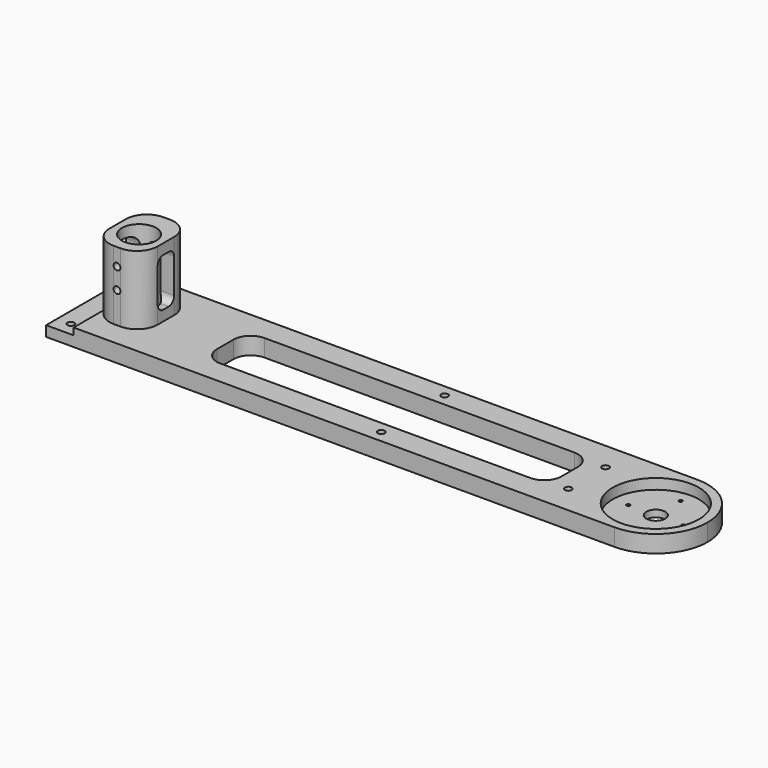
from build123d import *

# Parameters (mm, degrees)
F0_W      = 180
F0_H      = 30
F0_R      = 1
F0_W_2    = 100
F0_H_2    = 16
F1_DEPTH  = 5
F2_R      = 12.5
F2_R_2    = 0.5
F2_R_3    = 2.75
F3_DEPTH  = 3
F4_DEPTH  = 25
F5_R      = 14.99999
F2_R_4    = 5
F6_DEPTH  = 25
F7_R      = 5
F2_W      = 14
F2_H      = 18
F8_DEPTH  = 20
F9_R      = 6
F2_R_5    = 1
F10_DEPTH = 2
F11_W     = 6
F11_H     = 14
F12_DEPTH = 25
F13_R     = 2
F15_DEPTH = 25


# Not quite as in the source:
# - a fillet or chamfer is up to 0.001 mm smaller than in the source, because OpenCascade refuses the exact size


with BuildPart() as f1:
    # F0 (on Top) → F1 (new body)
    with BuildSketch(Plane.XY):
        with Locations((10, -11.8972941886)):
            Rectangle(F0_W, F0_H)
        with Locations((-76, -22.8972941886)):
            Circle(F0_R, mode=Mode.SUBTRACT)
        with Locations((14.5, -23.3972941886)):
            Circle(F0_R, mode=Mode.SUBTRACT)
        with Locations((10, -11.8972941886)):
            Rectangle(F0_W_2, F0_H_2, mode=Mode.SUBTRACT)
        with Locations((65, -18.6472941886)):
            Circle(F0_R, mode=Mode.SUBTRACT)
        with Locations((-76, -0.8972941886)):
            Circle(F0_R, mode=Mode.SUBTRACT)
        with Locations((65, -5.1472941886)):
            Circle(F0_R, mode=Mode.SUBTRACT)
        with Locations((14.5, -0.3972941886)):
            Circle(F0_R, mode=Mode.SUBTRACT)
    extrude(amount=F1_DEPTH)

    # F2 (on face) → F3 (cut)
    with BuildSketch(Plane.XY.offset(5)):
        with Locations((85, -11.8972941886)):
            Circle(F2_R)
        with Locations((85, -20.8972941886)):
            Circle(F2_R_2, mode=Mode.SUBTRACT)
        with Locations((85, -11.8972941886)):
            Circle(F2_R_3, mode=Mode.SUBTRACT)
        with Locations((77, -11.8972941886)):
            Circle(F2_R_2, mode=Mode.SUBTRACT)
        with Locations((93, -11.8972941886)):
            Circle(F2_R_2, mode=Mode.SUBTRACT)
        with Locations((85, -2.8972941886)):
            Circle(F2_R_2, mode=Mode.SUBTRACT)
    extrude(amount=-F3_DEPTH, mode=Mode.SUBTRACT)

    # F2 (on face) → F4 (cut)
    with BuildSketch(Plane.XY.offset(5)):
        with Locations((85, -11.8972941886)):
            Circle(F2_R_3)
        with Locations((85, -2.8972941886)):
            Circle(F2_R_2)
        with Locations((77, -11.8972941886)):
            Circle(F2_R_2)
        with Locations((85, -20.8972941886)):
            Circle(F2_R_2)
        with Locations((93, -11.8972941886)):
            Circle(F2_R_2)
    extrude(amount=-F4_DEPTH, mode=Mode.SUBTRACT)

    # F5 (radius 15 in the source; OpenCascade refuses exactly that, so slightly less here)
    f5_edges = [f1.edges().sort_by_distance(p)[0] for p in [
        (100, 3.102706, 2.5),
        (100, -26.897294, 2.5),
    ]]
    fillet(f5_edges, radius=F5_R)

    # F2 (on face) → F6 (cut)
    with BuildSketch(Plane.XY.offset(5)):
        with Locations((-65, -11.8972941886)):
            Circle(F2_R_4)
    extrude(amount=-F6_DEPTH, mode=Mode.SUBTRACT)

    # F7
    f7_edges = [f1.edges().sort_by_distance(p)[0] for p in [
        (-40, -3.897294, 2.5),
        (-40, -19.897294, 2.5),
        (60, -3.897294, 2.5),
        (60, -19.897294, 2.5),
    ]]
    fillet(f7_edges, radius=F7_R)

    # F2 (on face) → F8 (join)
    with BuildSketch(Plane.XY.offset(5)):
        with Locations((-65, -10.8972941886)):
            Rectangle(F2_W, F2_H)
        with Locations((-65, -11.8972941886)):
            Circle(F2_R_4, mode=Mode.SUBTRACT)
    extrude(amount=F8_DEPTH)

    # F9
    f9_edges = [f1.edges().sort_by_distance(p)[0] for p in [
        (-72, -19.897294, 15),
        (-58, -19.897294, 15),
        (-72, -1.897294, 15),
        (-58, -1.897294, 15),
    ]]
    fillet(f9_edges, radius=F9_R)

    # F2 (on face) → F10 (cut)
    with BuildSketch(Plane.XY.offset(5)):
        Polygon((-72, -19.8972941886), (-72, -1.8972941886), (-72, 3.1027058114), (-80, 3.1027058114), (-80, -26.8972941886), (-72, -26.8972941886), align=None)
        with Locations((-76, -22.8972941886)):
            Circle(F2_R_5, mode=Mode.SUBTRACT)
        with Locations((-76, -0.8972941886)):
            Circle(F2_R_5, mode=Mode.SUBTRACT)
    extrude(amount=-F10_DEPTH, mode=Mode.SUBTRACT)

    # F11 (on face) → F12 (cut)
    with BuildSketch(Plane.YZ.offset(-58)):
        with Locations((-10.8972941886, 15)):
            Rectangle(F11_W, F11_H)
    extrude(amount=-F12_DEPTH, mode=Mode.SUBTRACT)

    # F13
    f13_edges = [f1.edges().sort_by_distance(p)[0] for p in [
        (-59.208712, -13.897294, 8),
        (-60, -7.897294, 8),
        (-60, -7.897294, 22),
        (-59.208712, -13.897294, 22),
        (-70.791288, -13.897294, 8),
        (-70, -7.897294, 8),
        (-70, -7.897294, 22),
        (-70.791288, -13.897294, 22),
    ]]
    fillet(f13_edges, radius=F13_R)

    # F14 (on face) → F15 (cut)
    with BuildSketch(Plane(origin=(0, -1.8972941886, 0), x_dir=(-1, 0, 0), z_dir=(0, 1, 0))):
        with BuildLine():
            ThreePointArc((64, 20), (65, 19), (66, 20))
            ThreePointArc((66, 20), (65, 21), (64, 20))
        make_face()
        with BuildLine():
            ThreePointArc((64, 14), (65, 13), (66, 14))
            ThreePointArc((66, 14), (65, 15), (64, 14))
        make_face()
    extrude(amount=-F15_DEPTH, mode=Mode.SUBTRACT)


solid = f1.part
